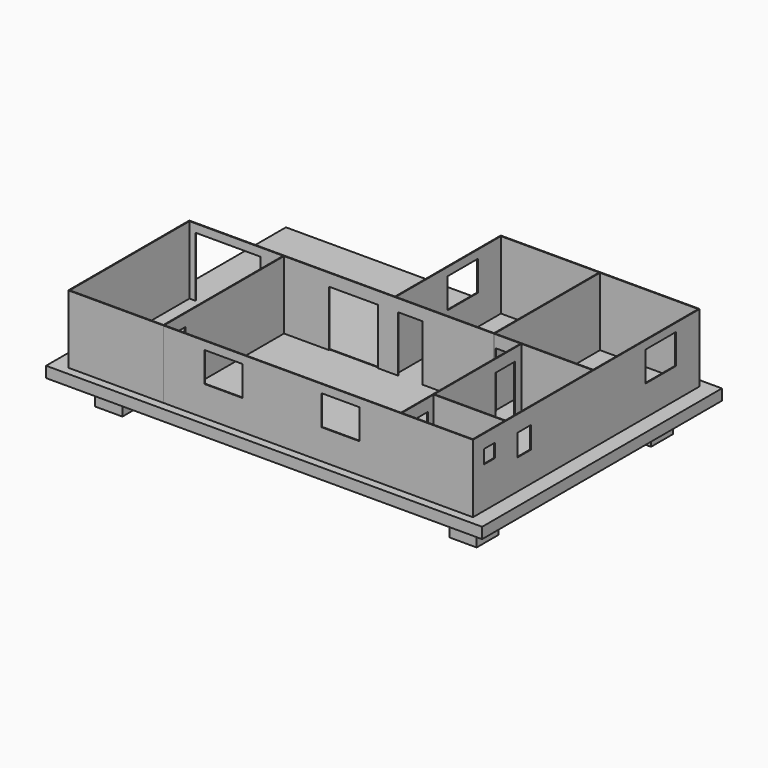
from build123d import *

# Parameters (mm, degrees)
F0_W      = 330
F0_H      = 555
F1_DEPTH  = 250
F3_DEPTH  = 250
F4_W      = 1600
F4_H      = 1100
F5_DEPTH  = 40
F6_W      = 350
F6_H      = 555
F7_DEPTH  = 250
F8_W      = 344
F8_H      = 549
F9_DEPTH  = 250
F10_W     = 240
F10_H     = 220
F11_DEPTH = 72
F12_W     = 90
F12_H     = 205
F13_DEPTH = 25
F14_W     = 730
F14_H     = 488
F15_DEPTH = 250
F16_W     = 724
F16_H     = 482
F17_DEPTH = 250
F18_W     = 3
F18_H     = 488
F19_DEPTH = 250
F20_W     = 474.8138537626
F20_H     = 317.8651188746
F21_DEPTH = 2
F22_W     = 3
F22_H     = 145.998
F22_W_2   = 260.499
F22_H_2   = 3
F23_DEPTH = 250
F24_W     = 90
F24_H     = 205
F25_DEPTH = 25
F26_W     = 90
F26_H     = 205
F27_DEPTH = 25
F28_W     = 180
F28_H     = 205
F29_DEPTH = 25
F30_W     = 140
F30_H     = 110
F31_DEPTH = 25
F32_W     = 140
F32_H     = 110
F32_W_2   = 50
F32_H_2   = 50
F32_W_3   = 60
F32_H_3   = 80
F33_DEPTH = 25
F34_W     = 140
F34_H     = 110
F35_DEPTH = 25
F36_W     = 100
F36_H     = 100
F37_DEPTH = 100
F38_W     = 400
F38_H     = 400
F39_DEPTH = 100
F40_W     = 340
F40_H     = 340
F41_DEPTH = 100


with BuildPart() as f1:
    # F0 (on Top) → F1 (new body)
    with BuildSketch(Plane.XY):
        Polygon((0, 277.2738870707), (0, -277.7261129293), (1155, -277.7261129293), (1155, 762.2738870707), (425, 762.2738870707), (425, 277.2738870707), align=None)
        with Locations((-165, -0.2261129293)):
            Rectangle(F0_W, F0_H)
    extrude(amount=F1_DEPTH)

    # F2 (on face) → F3 (cut)
    with BuildSketch(Plane.XY.offset(250)):
        Polygon((428, 274.2738870707), (-327, 274.2738870707), (-327, -274.7261129293), (1152, -274.7261129293), (1152, 759.2738870707), (428, 759.2738870707), align=None)
    extrude(amount=-F3_DEPTH, mode=Mode.SUBTRACT)


with BuildPart() as f5:
    # F4 (on face) → F5 (new body)
    with BuildSketch(Plane(origin=(0, 0, 0), x_dir=(1, 0, 0), z_dir=(0, 0, -1))):
        with Locations((412.5, -242.2738870707)):
            Rectangle(F4_W, F4_H)
    extrude(amount=F5_DEPTH)

    # F20 (on face) → F21 (join)
    with BuildSketch(Plane.XY):
        with Locations((186.5930731187, 437.206446508)):
            Rectangle(F20_W, F20_H)
    extrude(amount=F21_DEPTH)

    # F36 (on face) → F37 (join)
    with BuildSketch(Plane(origin=(0, 0, -40), x_dir=(1, 0, 0), z_dir=(0, 0, -1))):
        with Locations((-237.5, 157.7261129293)):
            Rectangle(F36_W, F36_H)
        with Locations((1062.5, 157.7261129293)):
            Rectangle(F36_W, F36_H)
        with Locations((1062.5, -642.2738870707)):
            Rectangle(F36_W, F36_H)
        with Locations((-237.5, -642.2738870707)):
            Rectangle(F36_W, F36_H)
    extrude(amount=F37_DEPTH)

    # F38 (on face) → F39 (join)
    with BuildSketch(Plane(origin=(0, 0, -40), x_dir=(1, 0, 0), z_dir=(0, 0, -1))):
        with Locations((412.5, -242.2738870707)):
            Rectangle(F38_W, F38_H)
    extrude(amount=F39_DEPTH)

    # F40 (on face) → F41 (cut)
    with BuildSketch(Plane(origin=(0, 0, -140), x_dir=(1, 0, 0), z_dir=(0, 0, -1))):
        with Locations((412.5, -242.2738870707)):
            Rectangle(F40_W, F40_H)
    extrude(amount=-F41_DEPTH, mode=Mode.SUBTRACT)


with BuildPart() as f7:
    # F6 (on face) → F7 (new body)
    with BuildSketch(Plane.XY.offset(250)):
        with Locations((-155, -0.2261129293)):
            Rectangle(F6_W, F6_H)
    extrude(amount=-F7_DEPTH)

    # F8 (on face) → F9 (cut)
    with BuildSketch(Plane.XY.offset(250)):
        with Locations((-155, -0.2261129293)):
            Rectangle(F8_W, F8_H)
    extrude(amount=-F9_DEPTH, mode=Mode.SUBTRACT)


with BuildPart() as f11_tool:
    # F10 (on face) → F11 (new body)
    with BuildSketch(Plane.XZ.offset(-274.2738870707)):
        with Locations((-185.4338693619, 110)):
            Rectangle(F10_W, F10_H)
    extrude(amount=-F11_DEPTH)


with BuildPart() as f1_1:
    add(f1.part)

    # F11: cut by f11_tool
    add(f11_tool.part, mode=Mode.SUBTRACT)

    # F14 (on face) → F15 (join)
    with BuildSketch(Plane.XY.offset(250)):
        with Locations((790, 518.2738870707)):
            Rectangle(F14_W, F14_H)
    extrude(amount=-F15_DEPTH)

    # F16 (on face) → F17 (cut)
    with BuildSketch(Plane.XY.offset(250)):
        with Locations((790, 518.2738870707)):
            Rectangle(F16_W, F16_H)
    extrude(amount=-F17_DEPTH, mode=Mode.SUBTRACT)

    # F26 (on face) → F27 (cut)
    with BuildSketch(Plane.XZ.offset(-274.2738870707)):
        with Locations((483, 102.5)):
            Rectangle(F26_W, F26_H)
        with Locations((840.5, 102.5)):
            Rectangle(F26_W, F26_H)
    extrude(amount=-F27_DEPTH, mode=Mode.SUBTRACT)

    # F28 (on face) → F29 (cut)
    with BuildSketch(Plane(origin=(0, 277.2738870707, 0), x_dir=(-1, 0, 0), z_dir=(0, 1, 0))):
        with Locations((-275, 102.5)):
            Rectangle(F28_W, F28_H)
    extrude(amount=-F29_DEPTH, mode=Mode.SUBTRACT)

    # F30 (on face) → F31 (cut)
    with BuildSketch(Plane(origin=(425, 0, 0), x_dir=(0, -1, 0), z_dir=(-1, 0, 0))):
        with Locations((-583.8110649586, 165)):
            Rectangle(F30_W, F30_H)
    extrude(amount=-F31_DEPTH, mode=Mode.SUBTRACT)

    # F32 (on face) → F33 (cut)
    with BuildSketch(Plane.YZ.offset(1155)):
        with Locations((583.5238695145, 165)):
            Rectangle(F32_W, F32_H)
        with Locations((-202.7261129293, 175)):
            Rectangle(F32_W_2, F32_H_2)
        with Locations((-42.3974481225, 150)):
            Rectangle(F32_W_3, F32_H_3)
    extrude(amount=-F33_DEPTH, mode=Mode.SUBTRACT)

    # F34 (on face) → F35 (cut)
    with BuildSketch(Plane.XZ.offset(277.7261129293)):
        with Locations((240, 165)):
            Rectangle(F34_W, F34_H)
        with Locations((668.5, 165)):
            Rectangle(F34_W, F34_H)
    extrude(amount=-F35_DEPTH, mode=Mode.SUBTRACT)


with BuildPart() as f7_1:
    add(f7.part)

    # F11: cut by f11_tool
    add(f11_tool.part, mode=Mode.SUBTRACT)

    # F12 (on face) → F13 (cut)
    with BuildSketch(Plane.YZ.offset(20)):
        with Locations((-222.7261129293, 102.5)):
            Rectangle(F12_W, F12_H)
    extrude(amount=-F13_DEPTH, mode=Mode.SUBTRACT)


with BuildPart() as f19:
    # F18 (on face) → F19 (new body)
    with BuildSketch(Plane.XY.offset(250)):
        with Locations((790, 518.2738870707)):
            Rectangle(F18_W, F18_H)
    extrude(amount=-F19_DEPTH)


with BuildPart() as f23:
    # F22 (on face) → F23 (new body)
    with BuildSketch(Plane.XY):
        Polygon((891.5, 274.2728870707), (888.5, 274.2728870707), (888.5, -128.7271129293), (891.5, -128.7271129293), (891.5, -125.7271129293), align=None)
        with Locations((890, -201.7261129293)):
            Rectangle(F22_W, F22_H)
        with Locations((1021.7495, -127.2271129293)):
            Rectangle(F22_W_2, F22_H_2)
    extrude(amount=F23_DEPTH)

    # F24 (on face) → F25 (cut)
    with BuildSketch(Plane(origin=(888.5, 0, 0), x_dir=(0, -1, 0), z_dir=(-1, 0, 0))):
        with Locations((199.7251129293, 102.5)):
            Rectangle(F24_W, F24_H)
        with Locations((-199.2728870707, 102.5)):
            Rectangle(F24_W, F24_H)
    extrude(amount=-F25_DEPTH, mode=Mode.SUBTRACT)


solid = Compound([f5.part, f1_1.part, f7_1.part, f19.part, f23.part])
